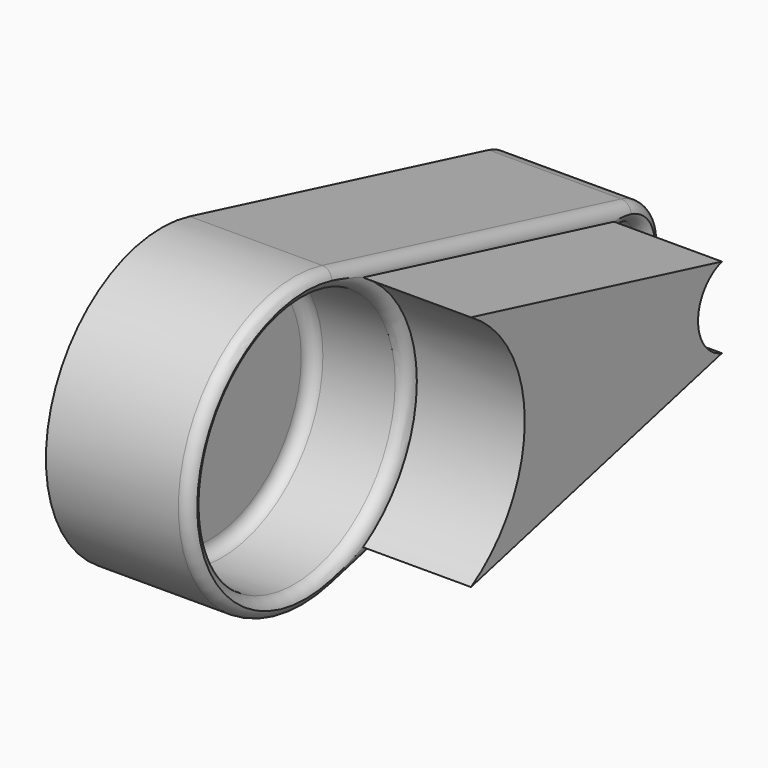
from build123d import *

# Parameters (mm, degrees)
F1_DEPTH = 76.2
F2_R     = 66.675
F2_R_2   = 15.875
F3_DEPTH = 50.8
F4_T     = -2.54
F5_F1_R  = 6.35
F5_F2_R  = 6.35
F5_F3_R  = 6.35
F6_DEPTH = 56.896
F7_DEPTH = 144.018


# Not quite as in the source:
# - a fillet or chamfer that OpenCascade refuses, or shapes differently, is made with other operations: its cross-section is extruded or revolved along the edge and cut away or added


with BuildPart() as f1:
    # F0 (on Right) → F1 (new body)
    with BuildSketch(Plane.YZ):
        with BuildLine():
            ThreePointArc((18.4812146278, -73.9248585111), (60.0612543768, -46.8944103565), (76.2, 0))
            ThreePointArc((76.2, 0), (60.0612543768, 46.8944103565), (18.4812146278, 73.9248585111))
            ThreePointArc((18.4812146278, 73.9248585111), (-76.2, 0), (18.4812146278, -73.9248585111))
        make_face()
        with BuildLine():
            ThreePointArc((18.4812146278, 73.9248585111), (60.0612543768, 46.8944103565), (76.2, 0))
            ThreePointArc((76.2, 0), (60.0612543768, -46.8944103565), (18.4812146278, -73.9248585111))
            Line((18.4812146278, -73.9248585111), (215.6141706573, -24.6416195037))
            ThreePointArc((215.6141706573, -24.6416195037), (184.0537657814, 0), (215.6141706573, 24.6416195037))
            Line((215.6141706573, 24.6416195037), (18.4812146278, 73.9248585111))
        make_face()
        with BuildLine():
            ThreePointArc((234.8537657814, 0), (229.474183907, 15.6314701188), (215.6141706573, 24.6416195037))
            ThreePointArc((215.6141706573, 24.6416195037), (184.0537657814, 0), (215.6141706573, -24.6416195037))
            ThreePointArc((215.6141706573, -24.6416195037), (229.474183907, -15.6314701188), (234.8537657814, 0))
        make_face()
    extrude(amount=F1_DEPTH)

    # F2 (on face) → F3 (cut)
    with BuildSketch(Plane.YZ.offset(76.2)):
        Circle(F2_R)
        with Locations((209.4537657814, 0)):
            Circle(F2_R_2)
    extrude(amount=-F3_DEPTH, mode=Mode.SUBTRACT)

    # F4
    f4_openings = [f1.faces().sort_by_distance(p)[0] for p in [
        (0, 57.51924, 0),
    ]]
    offset(amount=F4_T, openings=f4_openings, kind=Kind.INTERSECTION)

    # F5: fillet of radius 6.35 on 8 edges, made by hand

    # F5_f1
    f5_f1_edges = [f1.edges().sort_by_distance(p)[0] for p in [
        (76.2, -76.2, 0),
        (76.2, 117.0476926425, 49.2832390074),
        (76.2, 117.0476926425, -49.2832390074),
        (76.2, 234.8537657814, 0),
    ]]
    fillet(f5_f1_edges, radius=F5_F1_R)

    # F5_f2
    f5_f2_edges = [f1.edges().sort_by_distance(p)[0] for p in [
        (25.4, -66.675, 0),
    ]]
    fillet(f5_f2_edges, radius=F5_F2_R)

    # F5_f3
    f5_f3_edges = [f1.edges().sort_by_distance(p)[0] for p in [
        (25.4, 193.5787657814, 0),
    ]]
    fillet(f5_f3_edges, radius=F5_F3_R)

    # F5_s4 → F5_t5 (revolve, cut)
    with BuildSketch(Plane.XY):
        with BuildLine():
            ThreePointArc((76.2, 73.025), (74.3401280605, 68.5348719395), (69.85, 66.675))
            Line((69.85, 66.675), (69.85, 66.548))
            Line((69.85, 66.548), (76.327, 66.548))
            Line((76.327, 66.548), (76.327, 73.025))
            Line((76.327, 73.025), (76.2, 73.025))
        make_face()
    revolve(axis=Axis((76.2, 0, 0), (1, 0, 0)), mode=Mode.SUBTRACT)

    # F5_s6 → F5_t7 (revolve, cut)
    with BuildSketch(Plane.XY):
        with BuildLine():
            ThreePointArc((69.85, 225.3287657814), (74.3401280605, 227.1886377208), (76.2, 231.6787657814))
            Line((76.2, 231.6787657814), (76.327, 231.6787657814))
            Line((76.327, 231.6787657814), (76.327, 225.2017657814))
            Line((76.327, 225.2017657814), (69.85, 225.2017657814))
            Line((69.85, 225.2017657814), (69.85, 225.3287657814))
        make_face()
    revolve(axis=Axis((76.2, 209.4537657814, 0), (1, 0, 0)), mode=Mode.SUBTRACT)

    # F6 (add): a face of the model
    f6_faces = [f1.faces().sort_by_distance(p)[0] for p in [
        (76.2, 119.1189366743, 0),
    ]]
    extrude(f6_faces, amount=F6_DEPTH)

    # F7 (add): a face of the model
    f7_faces = [f1.faces().sort_by_distance(p)[0] for p in [
        (133.096, 119.1189366743, 0),
    ]]
    extrude(f7_faces, amount=-F7_DEPTH)


solid = f1.part
